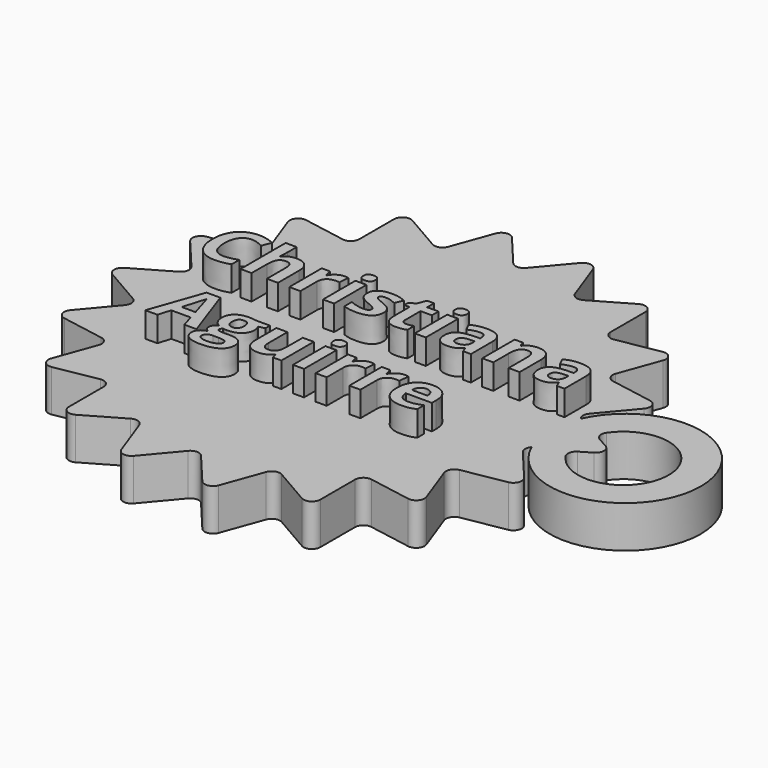
from build123d import *

# Parameters (mm, degrees)
F1_DEPTH      = 5
F2_R          = 1
F3_R          = 1
F4_R          = 9.02426598
F5_DEPTH      = 5
F7_DEPTH      = 5
F8_R          = 1
F10_DEPTH     = 4.5
F11_R         = 7.0893465871
F11_R_2       = 5.3736476411
F12_DEPTH     = 4.5
F13_TEXT_SIZE = 8.8585401864
F14_DEPTH     = 3


# Not quite as in the source:
# - a feature names something its author has since deleted; it is built from what else it names
# - Text() gives the source's letters only with a copy of the font that has no kerning and outlines rounded to 1/6400 em; it was checked with that copy


with BuildPart() as f1:
    # F0 (on Top) → F1 (new body)
    with BuildSketch(Plane.XY):
        Polygon((-69.4327632519, 10.2606042998), (-64.2233179219, 4.0522291123), (-71.2419846284, 0), (-64.2233179219, -4.0522291123), (-69.4327632519, -10.2606042998), (-61.4514299584, -11.6679287015), (-64.2233179219, -19.2836282906), (-56.2419846284, -17.8763038889), (-56.2419846284, -25.9807621135), (-49.2233179219, -21.9285330012), (-46.4514299584, -29.5442325904), (-41.2419846284, -23.3358574029), (-36.0325392983, -29.5442325904), (-33.2606513348, -21.9285330012), (-26.2419846284, -25.9807621135), (-26.2419846284, -17.8763038889), (-18.2606513348, -19.2836282906), (-21.0325392984, -11.6679287015), (-13.0512060048, -10.2606042998), (-18.2606513348, -4.0522291123), (-11.2419846284, 0), (-18.2606513348, 4.0522291123), (-13.0512060048, 10.2606042998), (-21.0325392984, 11.6679287015), (-18.2606513348, 19.2836282906), (-26.2419846284, 17.8763038889), (-26.2419846284, 25.9807621135), (-33.2606513348, 21.9285330012), (-36.0325392984, 29.5442325904), (-41.2419846284, 23.3358574029), (-46.4514299584, 29.5442325904), (-49.2233179219, 21.9285330012), (-56.2419846284, 25.9807621135), (-56.2419846284, 17.8763038889), (-64.2233179219, 19.2836282906), (-61.4514299584, 11.6679287015), align=None)
    extrude(amount=F1_DEPTH)

    # F2
    f2_edges = [f1.edges().sort_by_distance(p)[0] for p in [
        (-49.223318, -21.928533, 2.5),
        (-56.241985, -17.876304, 2.5),
        (-61.45143, -11.667929, 2.5),
        (-64.223318, -4.052229, 2.5),
        (-64.223318, 4.052229, 2.5),
        (-61.45143, 11.667929, 2.5),
        (-56.241985, 17.876304, 2.5),
        (-49.223318, 21.928533, 2.5),
        (-41.241985, 23.335857, 2.5),
        (-33.260651, 21.928533, 2.5),
        (-41.241985, -23.335857, 2.5),
        (-33.260651, -21.928533, 2.5),
        (-26.241985, -17.876304, 2.5),
        (-21.032539, -11.667929, 2.5),
        (-26.241985, 17.876304, 2.5),
        (-21.032539, 11.667929, 2.5),
        (-18.260651, 4.052229, 2.5),
        (-18.260651, -4.052229, 2.5),
    ]]
    fillet(f2_edges, radius=F2_R)

    # F3
    f3_edges = [f1.edges().sort_by_distance(p)[0] for p in [
        (-36.032539, 29.544233, 2.5),
        (-26.241985, 25.980762, 2.5),
        (-18.260651, 19.283628, 2.5),
        (-13.051206, 10.260604, 2.5),
        (-11.241985, 0, 2.5),
        (-13.051206, -10.260604, 2.5),
        (-56.241985, 25.980762, 2.5),
        (-46.45143, 29.544233, 2.5),
        (-64.223318, 19.283628, 2.5),
        (-69.432763, 10.260604, 2.5),
        (-71.241985, 0, 2.5),
        (-69.432763, -10.260604, 2.5),
        (-64.223318, -19.283628, 2.5),
        (-56.241985, -25.980762, 2.5),
        (-46.45143, -29.544233, 2.5),
        (-36.032539, -29.544233, 2.5),
        (-26.241985, -25.980762, 2.5),
        (-18.260651, -19.283628, 2.5),
    ]]
    fillet(f3_edges, radius=F3_R)

    # F4 (on Top) → F5 (join, through all)
    with BuildSketch(Plane.XY):
        with Locations((-9.2419846284, 0)):
            Circle(F4_R)
    extrude(amount=F5_DEPTH)

    # F6 (on face) → F7 (cut, through all)
    with BuildSketch(Plane.XY.offset(5)):
        with BuildLine():
            ThreePointArc((-14.3705448136, -2.1852792706), (-3.981082649, -0.0942598595), (-14.3705448136, 1.9967595517))
            Line((-14.3705448136, 1.9967595517), (-10.7515631244, 0))
            Line((-10.7515631244, 0), (-14.3705448136, -2.1852792706))
        make_face()
    extrude(amount=-F7_DEPTH, mode=Mode.SUBTRACT)

    # F8
    f8_edges = [f1.edges().sort_by_distance(p)[0] for p in [
        (-10.751563, 0, 2.5),
        (-14.370545, -2.185279, 2.5),
        (-14.370545, 1.99676, 2.5),
    ]]
    fillet(f8_edges, radius=F8_R)

    # F9 (on face) → F10 (cut)
    with BuildSketch(Plane.XY):
        with BuildLine():
            ThreePointArc((-35.3777156799, -4.6599307489), (-35.5753046169, -4.908160303), (-35.7829730175, -5.1480209603))
            Line((-35.7829730175, -5.1480209603), (-21.9766725259, -17.609254409))
            Line((-21.9766725259, -17.609254409), (-20.5904544794, -15.9396992978))
            Line((-20.5904544794, -15.9396992978), (-35.3777156799, -4.6599307489))
        make_face()
        with BuildLine():
            Line((-35.0430152336, -4.1849240607), (-22.1269458204, -12.5734481191))
            Line((-22.1269458204, -12.5734481191), (-20.8090839907, -10.2629405882))
            Line((-20.8090839907, -10.2629405882), (-34.6043804511, -3.4158988524))
            ThreePointArc((-34.6043804511, -3.4158988524), (-34.8126121734, -3.8067344742), (-35.0430152336, -4.1849240607))
        make_face()
        with BuildLine():
            ThreePointArc((-34.1823081919, -2.3833949122), (-34.2698744439, -2.6366901562), (-34.3662212872, -2.8867773708))
            Line((-34.3662212872, -2.8867773708), (-17.1305497448, -9.8744736155))
            Line((-17.1305497448, -9.8744736155), (-16.3989523541, -7.8314905025))
            Line((-16.3989523541, -7.8314905025), (-19.4509472573, -6.8787666419))
            Line((-19.4509472573, -6.8787666419), (-34.1823081919, -2.3833949122))
        make_face()
        with BuildLine():
            Line((-34.0002869576, -1.7286818538), (-18.9941076397, -5.1937600989))
            Line((-18.9941076397, -5.1937600989), (-18.54596272, -2.5718579299))
            Line((-18.54596272, -2.5718579299), (-33.8511272013, -0.8560126092))
            ThreePointArc((-33.8511272013, -0.8560126092), (-33.9131273587, -1.2944974025), (-34.0002869576, -1.7286818538))
        make_face()
        with BuildLine():
            ThreePointArc((-33.8115942061, 0.3570473634), (-33.8033972316, 0.0398847724), (-33.8083009973, -0.2773458261))
            Line((-33.8083009973, -0.2773458261), (-15.2221347635, -0.9486855723))
            Line((-15.2221347635, -0.9486855723), (-15.2333994712, 1.2213116278))
            Line((-15.2333994712, 1.2213116278), (-33.8115942061, 0.3570473634))
        make_face()
        with BuildLine():
            Line((-33.8605272028, 0.9360648973), (-18.5742046736, 2.812372041))
            Line((-18.5742046736, 2.812372041), (-19.0498295551, 5.4294287513))
            Line((-19.0498295551, 5.4294287513), (-34.0188333405, 1.807121388))
            ThreePointArc((-34.0188333405, 1.807121388), (-33.9271237992, 1.3738751607), (-33.8605272028, 0.9360648973))
        make_face()
        with BuildLine():
            ThreePointArc((-34.3965754224, 2.9605459736), (-34.2803967911, 2.6653141576), (-34.1765055688, 2.3655377184))
            Line((-34.1765055688, 2.3655377184), (-16.481610594, 8.0915279521))
            Line((-16.481610594, 8.0915279521), (-17.2343787101, 10.1268055511))
            Line((-17.2343787101, 10.1268055511), (-34.3965754224, 2.9605459736))
        make_face()
        with BuildLine():
            Line((-34.6405930582, 3.4879084069), (-20.9178834168, 10.4792906065))
            Line((-20.9178834168, 10.4792906065), (-22.2599107194, 12.7758461952))
            Line((-22.2599107194, 12.7758461952), (-35.0872710335, 4.2522898756))
            ThreePointArc((-35.0872710335, 4.2522898756), (-34.8529133175, 3.8765381033), (-34.6405930582, 3.4879084069))
        make_face()
        with BuildLine():
            ThreePointArc((-35.8367269225, 5.2069590463), (-35.6265794919, 4.9692673195), (-35.4264240963, 4.7231025025))
            Line((-35.4264240963, 4.7231025025), (-20.7570658633, 16.1557837872))
            Line((-20.7570658633, 16.1557837872), (-22.1605424433, 17.8108572693))
            Line((-22.1605424433, 17.8108572693), (-35.8367269225, 5.2069590463))
        make_face()
        with BuildLine():
            Line((-36.2463970692, 5.6190586866), (-25.742461624, 16.882252067))
            Line((-25.742461624, 16.882252067), (-27.7890230487, 18.5813080366))
            Line((-27.7890230487, 18.5813080366), (-36.927570926, 6.184569447))
            ThreePointArc((-36.927570926, 6.184569447), (-36.5788320346, 5.911633339), (-36.2463970692, 5.6190586866))
        make_face()
        with BuildLine():
            ThreePointArc((-37.958345181, 6.8253360115), (-37.6795758328, 6.6738535042), (-37.4072979585, 6.5109914192))
            Line((-37.4072979585, 6.5109914192), (-27.5328175668, 22.2714136636))
            Line((-27.5328175668, 22.2714136636), (-29.4177226221, 23.3466567405))
            Line((-29.4177226221, 23.3466567405), (-37.958345181, 6.8253360115))
        make_face()
        with BuildLine():
            Line((-38.4842555729, 7.0724675602), (-32.4660239601, 21.2489647728))
            Line((-32.4660239601, 21.2489647728), (-34.9702739951, 22.1455898979))
            Line((-34.9702739951, 22.1455898979), (-39.3177656909, 7.3708986687))
            ThreePointArc((-39.3177656909, 7.3708986687), (-38.8967086813, 7.2336983476), (-38.4842555729, 7.0724675602))
        make_face()
        with BuildLine():
            ThreePointArc((-40.5055317243, 7.6204767225), (-40.191764156, 7.5734744606), (-39.8802045331, 7.5135586787))
            Line((-39.8802045331, 7.5135586787), (-35.9916100498, 25.7007823611))
            Line((-35.9916100498, 25.7007823611), (-38.1305962124, 26.0665048489))
            Line((-38.1305962124, 26.0665048489), (-40.5055317243, 7.6204767225))
        make_face()
        with BuildLine():
            Line((-41.0842498064, 7.6728324676), (-40.2776095782, 23.0527387256))
            Line((-40.2776095782, 23.0527387256), (-42.9374987105, 23.0387867834))
            Line((-42.9374987105, 23.0387867834), (-41.9695625642, 7.668188728))
            ThreePointArc((-41.9695625642, 7.668188728), (-41.5269731258, 7.6832725775), (-41.0842498064, 7.6728324676))
        make_face()
        with BuildLine():
            ThreePointArc((-43.1710582627, 7.4964754745), (-42.8601374738, 7.5596226245), (-42.5468747909, 7.6098798733))
            Line((-42.5468747909, 7.6098798733), (-45.1131881003, 26.0302574027))
            Line((-45.1131881003, 26.0302574027), (-47.2482620709, 25.6423477718))
            Line((-47.2482620709, 25.6423477718), (-43.1710582627, 7.4964754745))
        make_face()
        with BuildLine():
            Line((-43.7327820934, 7.3477405404), (-48.235025966, 22.0760121659))
            Line((-48.235025966, 22.0760121659), (-50.7297323105, 21.1531659665))
            Line((-50.7297323105, 21.1531659665), (-44.5631157065, 7.0405820563))
            ThreePointArc((-44.5631157065, 7.0405820563), (-44.1523766576, 7.2061307415), (-43.7327820934, 7.3477405404))
        make_face()
        with BuildLine():
            ThreePointArc((-45.6334229567, 6.468288648), (-45.362850583, 6.6339687317), (-45.085668943, 6.7883372453))
            Line((-45.085668943, 6.7883372453), (-53.7973547852, 23.2200992358))
            Line((-53.7973547852, 23.2200992358), (-55.6709951327, 22.1253451128))
            Line((-55.6709951327, 22.1253451128), (-45.6334229567, 6.468288648))
        make_face()
        with BuildLine():
            Line((-46.1104003519, 6.1364026629), (-55.3784912683, 18.4365927318))
            Line((-55.3784912683, 18.4365927318), (-57.4071164218, 16.7161611466))
            Line((-57.4071164218, 16.7161611466), (-46.7856043321, 5.5637772807))
            ThreePointArc((-46.7856043321, 5.5637772807), (-46.4562568639, 5.8598231869), (-46.1104003519, 6.1364026629))
        make_face()
        with BuildLine():
            ThreePointArc((-47.5956282836, 4.6599307489), (-47.3980393467, 4.908160303), (-47.190370946, 5.1480209603))
            Line((-47.190370946, 5.1480209603), (-60.9966714376, 17.609254409))
            Line((-60.9966714376, 17.609254409), (-62.3828894841, 15.9396992978))
            Line((-62.3828894841, 15.9396992978), (-47.5956282836, 4.6599307489))
        make_face()
        with BuildLine():
            Line((-47.93032873, 4.1849240607), (-60.8463981431, 12.5734481191))
            Line((-60.8463981431, 12.5734481191), (-62.1642599729, 10.2629405882))
            Line((-62.1642599729, 10.2629405882), (-48.3689635124, 3.4158988524))
            ThreePointArc((-48.3689635124, 3.4158988524), (-48.1607317901, 3.8067344742), (-47.93032873, 4.1849240607))
        make_face()
        with BuildLine():
            ThreePointArc((-48.821003322, 2.2895164282), (-48.7202299636, 2.590355305), (-48.6071226764, 2.8867773708))
            Line((-48.6071226764, 2.8867773708), (-65.8427942188, 9.8744736155))
            Line((-65.8427942188, 9.8744736155), (-66.5743916094, 7.8314905025))
            Line((-66.5743916094, 7.8314905025), (-48.821003322, 2.2895164282))
        make_face()
        with BuildLine():
            Line((-48.973057006, 1.7286818538), (-63.9792363238, 5.1937600989))
            Line((-63.9792363238, 5.1937600989), (-64.4273812436, 2.5718579299))
            Line((-64.4273812436, 2.5718579299), (-49.1222167623, 0.8560126092))
            ThreePointArc((-49.1222167623, 0.8560126092), (-49.0602166048, 1.2944974025), (-48.973057006, 1.7286818538))
        make_face()
        Polygon((-49.1617497575, -0.3570473634), (-49.1650429663, 0.2773458261), (-67.7512092001, 0.9486855723), (-67.7399444924, -1.2213116278), align=None)
        with BuildLine():
            ThreePointArc((-48.5767685411, -2.9605459736), (-48.6929471725, -2.6653141576), (-48.7968383947, -2.3655377184))
            Line((-48.7968383947, -2.3655377184), (-66.4917333696, -8.0915279521))
            Line((-66.4917333696, -8.0915279521), (-65.7389652535, -10.1268055511))
            Line((-65.7389652535, -10.1268055511), (-48.5767685411, -2.9605459736))
        make_face()
        with BuildLine():
            Line((-49.1128167608, -0.9360648973), (-64.39913929, -2.812372041))
            Line((-64.39913929, -2.812372041), (-63.9235144085, -5.4294287513))
            Line((-63.9235144085, -5.4294287513), (-48.954510623, -1.807121388))
            ThreePointArc((-48.954510623, -1.807121388), (-49.0462201644, -1.3738751607), (-49.1128167608, -0.9360648973))
        make_face()
        with BuildLine():
            Line((-48.3327509053, -3.4879084069), (-62.0554605467, -10.4792906065))
            Line((-62.0554605467, -10.4792906065), (-60.7134332442, -12.7758461952))
            Line((-60.7134332442, -12.7758461952), (-47.88607293, -4.2522898756))
            ThreePointArc((-47.88607293, -4.2522898756), (-48.1204306461, -3.8765381033), (-48.3327509053, -3.4879084069))
        make_face()
        with BuildLine():
            ThreePointArc((-47.1366170411, -5.2069590463), (-47.3467644716, -4.9692673195), (-47.5469198672, -4.7231025025))
            Line((-47.5469198672, -4.7231025025), (-62.2162781003, -16.1557837872))
            Line((-62.2162781003, -16.1557837872), (-60.8128015203, -17.8108572693))
            Line((-60.8128015203, -17.8108572693), (-47.1366170411, -5.2069590463))
        make_face()
        with BuildLine():
            Line((-46.7269468943, -5.6190586866), (-57.2308823396, -16.882252067))
            Line((-57.2308823396, -16.882252067), (-55.1843209149, -18.5813080366))
            Line((-55.1843209149, -18.5813080366), (-46.0457730376, -6.184569447))
            ThreePointArc((-46.0457730376, -6.184569447), (-46.394511929, -5.911633339), (-46.7269468943, -5.6190586866))
        make_face()
        with BuildLine():
            ThreePointArc((-45.0149987825, -6.8253360115), (-45.2937681308, -6.6738535042), (-45.566046005, -6.5109914192))
            Line((-45.566046005, -6.5109914192), (-55.4405263967, -22.2714136636))
            Line((-55.4405263967, -22.2714136636), (-53.5556213415, -23.3466567405))
            Line((-53.5556213415, -23.3466567405), (-45.0149987825, -6.8253360115))
        make_face()
        with BuildLine():
            Line((-44.4890883907, -7.0724675602), (-50.5073200035, -21.2489647728))
            Line((-50.5073200035, -21.2489647728), (-48.0030699685, -22.1455898979))
            Line((-48.0030699685, -22.1455898979), (-43.6555782727, -7.3708986687))
            ThreePointArc((-43.6555782727, -7.3708986687), (-44.0766352823, -7.2336983476), (-44.4890883907, -7.0724675602))
        make_face()
        with BuildLine():
            ThreePointArc((-42.4678122393, -7.6204767225), (-42.7815798076, -7.5734744606), (-43.0931394305, -7.5135586787))
            Line((-43.0931394305, -7.5135586787), (-46.9817339137, -25.7007823611))
            Line((-46.9817339137, -25.7007823611), (-44.8427477512, -26.0665048489))
            Line((-44.8427477512, -26.0665048489), (-42.4678122393, -7.6204767225))
        make_face()
        with BuildLine():
            Line((-41.8890941571, -7.6728324676), (-42.6957343854, -23.0527387256))
            Line((-42.6957343854, -23.0527387256), (-40.0358452531, -23.0387867834))
            Line((-40.0358452531, -23.0387867834), (-41.0037813994, -7.668188728))
            ThreePointArc((-41.0037813994, -7.668188728), (-41.4463708377, -7.6832725775), (-41.8890941571, -7.6728324676))
        make_face()
        with BuildLine():
            ThreePointArc((-39.8022857009, -7.4964754745), (-40.1132064898, -7.5596226245), (-40.4264691727, -7.6098798733))
            Line((-40.4264691727, -7.6098798733), (-37.8601558633, -26.0302574027))
            Line((-37.8601558633, -26.0302574027), (-35.7250818926, -25.6423477718))
            Line((-35.7250818926, -25.6423477718), (-39.8022857009, -7.4964754745))
        make_face()
        with BuildLine():
            Line((-39.2405618701, -7.3477405404), (-34.7383179975, -22.0760121659))
            Line((-34.7383179975, -22.0760121659), (-32.2436116531, -21.1531659665))
            Line((-32.2436116531, -21.1531659665), (-38.4102282571, -7.0405820563))
            ThreePointArc((-38.4102282571, -7.0405820563), (-38.8209673059, -7.2061307415), (-39.2405618701, -7.3477405404))
        make_face()
        with BuildLine():
            ThreePointArc((-37.3399210068, -6.468288648), (-37.6104933805, -6.6339687317), (-37.8876750206, -6.7883372453))
            Line((-37.8876750206, -6.7883372453), (-29.1759891784, -23.2200992358))
            Line((-29.1759891784, -23.2200992358), (-27.3023488309, -22.1253451128))
            Line((-27.3023488309, -22.1253451128), (-37.3399210068, -6.468288648))
        make_face()
        with BuildLine():
            Line((-36.8629436116, -6.1364026629), (-27.5948526953, -18.4365927318))
            Line((-27.5948526953, -18.4365927318), (-25.5662275418, -16.7161611466))
            Line((-25.5662275418, -16.7161611466), (-36.1877396314, -5.5637772807))
            ThreePointArc((-36.1877396314, -5.5637772807), (-36.5170870997, -5.8598231869), (-36.8629436116, -6.1364026629))
        make_face()
    extrude(amount=F10_DEPTH, mode=Mode.SUBTRACT)

    # F11 (on face) → F12 (cut, through all)
    with BuildSketch(Plane.XY):
        with Locations((-41.4866719818, 0)):
            Circle(F11_R)
        with Locations((-41.4866719818, 0)):
            Circle(F11_R_2, mode=Mode.SUBTRACT)
    extrude(amount=F12_DEPTH, mode=Mode.SUBTRACT)

    # F13 (on face) → F14 (join)
    with BuildSketch(Plane.XY.offset(5)):
        with Locations((-63.8631587411, 2.95795153)):
            Text('Christiana', F13_TEXT_SIZE, font='Open Sans', font_style=FontStyle.BOLD, text_align=(TextAlign.LEFT, TextAlign.BOTTOM))
        with Locations((-59.259486138, -9.0896631236)):
            Text('Aguirre', F13_TEXT_SIZE, font='Open Sans', font_style=FontStyle.BOLD, text_align=(TextAlign.LEFT, TextAlign.BOTTOM))
    extrude(amount=F14_DEPTH)


solid = f1.part
